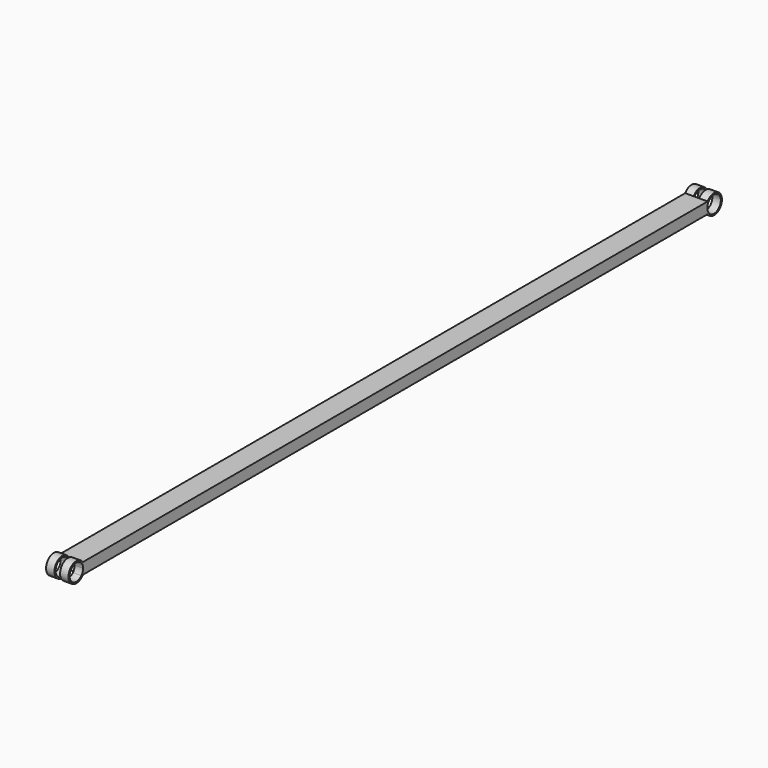
from build123d import *

# Parameters (mm, degrees)
F0_W     = 50.8
F0_H     = 25.4
F1_DEPTH = 1778
F6_DEPTH = 50.8
F4_R     = 22.225
F7_DEPTH = 12.7
F8_R     = 19.05
F9_DEPTH = 50.8


with BuildPart() as f1:
    # F0 (on Front) → F1 (new body)
    with BuildSketch(Plane.XZ):
        with Locations((25.4, 12.7)):
            Rectangle(F0_W, F0_H)
    extrude(amount=F1_DEPTH)

    # F5 (on face) → F6 (join)
    with BuildSketch(Plane.YZ.offset(50.8)):
        with BuildLine():
            ThreePointArc((36.0393014908, 12.7), (20.46971854, 33.9050948807), (-4.424684912, 25.4))
            Line((-4.424684912, 25.4), (0, 25.4))
            Line((0, 25.4), (0, 0))
            Line((0, 0), (-4.424684912, 0))
            ThreePointArc((-4.424684912, 0), (20.46971854, -8.5050948807), (36.0393014908, 12.7))
        make_face()
        with BuildLine():
            Line((-1777.6152698337, 25.4), (-1773.575315088, 25.4))
            ThreePointArc((-1773.575315088, 25.4), (-1814.0393014908, 12.7), (-1773.575315088, 0))
            Line((-1773.575315088, 0), (-1777.6152698337, 0))
            ThreePointArc((-1777.6152698337, 0), (-1810.8643014908, 12.7), (-1777.6152698337, 25.4))
        make_face()
    extrude(amount=-F6_DEPTH)

    # F4 (on offset) → F7 (cut)
    with BuildSketch(Plane.YZ.offset(31.75)):
        with Locations((-1791.8143014908, 12.7)):
            Circle(F4_R)
        with Locations((13.8143014908, 12.7)):
            Circle(F4_R)
    extrude(amount=-F7_DEPTH, mode=Mode.SUBTRACT)

    # F8 (on face) → F9 (cut)
    with BuildSketch(Plane.YZ.offset(50.8)):
        with BuildLine():
            ThreePointArc((-1777.6152698337, 0), (-1774.0183180525, 5.9025391898), (-1772.7643014908, 12.7))
            ThreePointArc((-1772.7643014908, 12.7), (-1774.0183180525, 19.4974608102), (-1777.6152698337, 25.4))
            Line((-1777.6152698337, 25.4), (-1778, 25.4))
            Line((-1778, 25.4), (-1778, 0))
            Line((-1778, 0), (-1777.6152698337, 0))
        make_face()
        with Locations((13.8143014908, 12.7)):
            Circle(F8_R)
    extrude(amount=-F9_DEPTH, mode=Mode.SUBTRACT)


solid = f1.part
